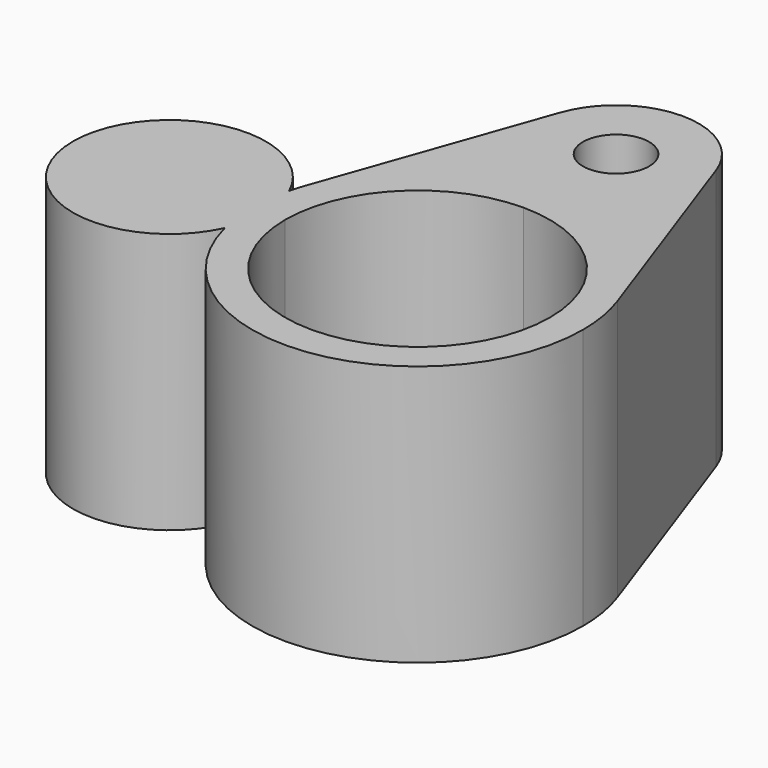
from build123d import *

# Parameters (mm, degrees)
F2_DEPTH = 34.036


# Not quite as in the source:
# - a variable given as a bare number and used for a length is read in inches; the dataset says mm whatever the document's units were


with BuildPart() as f2:
    # F1 (on Top) → F2 (new body)
    with BuildSketch(Plane.XY):
        with BuildLine():
            ThreePointArc((-20.9431391397, -5.2452857858), (2.6425107354, -21.4276745592), (21.59, 0))
            ThreePointArc((21.59, 0), (21.2790729029, 3.6509117207), (20.3552472078, 7.1966666667))
            ThreePointArc((20.3552472078, 7.1966666667), (12.4649923156, 17.6281611796), (9.2e-09, 21.59))
            Line((0, 21.59), (0, 17.272))
            ThreePointArc((0, 17.272), (12.2131483247, 12.2131483247), (17.272, 0))
            ThreePointArc((17.272, 0), (0, -17.272), (-17.272, 0))
            Line((-17.272, 0), (-19.7981337132, 0))
            ThreePointArc((-19.7981337132, 0), (-20.0877162422, -2.6844021868), (-20.9431391397, -5.2452857858))
        make_face()
        with BuildLine():
            ThreePointArc((9.2e-09, 21.59), (12.4649923156, 17.6281611796), (20.3552472078, 7.1966666667))
            Line((20.3552472078, 7.1966666667), (10.1776236039, 35.9833333333))
            ThreePointArc((10.1776236039, 35.9833333333), (10.6395364515, 34.2104558603), (10.795, 32.385))
            ThreePointArc((10.795, 32.385), (7.6332177062, 24.7517823004), (9.2e-09, 21.59))
        make_face()
        with BuildLine():
            ThreePointArc((-20.9431391397, 5.2452857858), (-44.9718662868, 0), (-20.9431391397, -5.2452857858))
            ThreePointArc((-20.9431391397, -5.2452857858), (-21.4276745592, -2.6425107354), (-21.59, 0))
            ThreePointArc((-21.59, 0), (-21.4276745592, 2.6425107354), (-20.9431391397, 5.2452857858))
        make_face()
        with BuildLine():
            ThreePointArc((-21.59, 0), (-21.4276745592, -2.6425107354), (-20.9431391397, -5.2452857858))
            ThreePointArc((-20.9431391397, -5.2452857858), (-20.0877162422, -2.6844021868), (-19.7981337132, 0))
            Line((-19.7981337132, 0), (-21.59, 0))
        make_face()
        with BuildLine():
            Line((0, 17.272), (0, 21.59))
            ThreePointArc((9.2e-09, 21.59), (-12.464992308, 17.6281611849), (-20.3552472078, 7.1966666667))
            ThreePointArc((-20.3552472078, 7.1966666667), (-20.6722313881, 6.2279169422), (-20.9431391397, 5.2452857858))
            ThreePointArc((-20.9431391397, 5.2452857858), (-20.0877162422, 2.6844021868), (-19.7981337132, 0))
            Line((-19.7981337132, 0), (-17.272, 0))
            ThreePointArc((-17.272, 0), (-12.2131483247, 12.2131483247), (0, 17.272))
        make_face()
        with BuildLine():
            ThreePointArc((-20.3552472078, 7.1966666667), (-12.464992308, 17.6281611849), (9.2e-09, 21.59))
            ThreePointArc((9.2e-09, 21.59), (-8.8140805884, 26.1525038403), (-10.1776236039, 35.9833333333))
            Line((-10.1776236039, 35.9833333333), (-20.3552472078, 7.1966666667))
        make_face()
        with BuildLine():
            ThreePointArc((-10.1776236039, 35.9833333333), (-8.8140805884, 26.1525038403), (9.2e-09, 21.59))
            ThreePointArc((9.2e-09, 21.59), (7.6332177062, 24.7517823004), (10.795, 32.385))
            ThreePointArc((10.795, 32.385), (10.6395364515, 34.2104558603), (10.1776236039, 35.9833333333))
            ThreePointArc((10.1776236039, 35.9833333333), (0, 43.18), (-10.1776236039, 35.9833333333))
        make_face()
        with BuildLine():
            ThreePointArc((4.318, 32.385), (3.0532870812, 29.3317129188), (0, 28.067))
            ThreePointArc((0, 28.067), (-3.0532870812, 35.4382870812), (4.318, 32.385))
        make_face(mode=Mode.SUBTRACT)
        with BuildLine():
            ThreePointArc((-20.9431391397, 5.2452857858), (-21.4276745592, 2.6425107354), (-21.59, 0))
            Line((-21.59, 0), (-19.7981337132, 0))
            ThreePointArc((-19.7981337132, 0), (-20.0877162422, 2.6844021868), (-20.9431391397, 5.2452857858))
        make_face()
    extrude(amount=F2_DEPTH)


solid = f2.part
